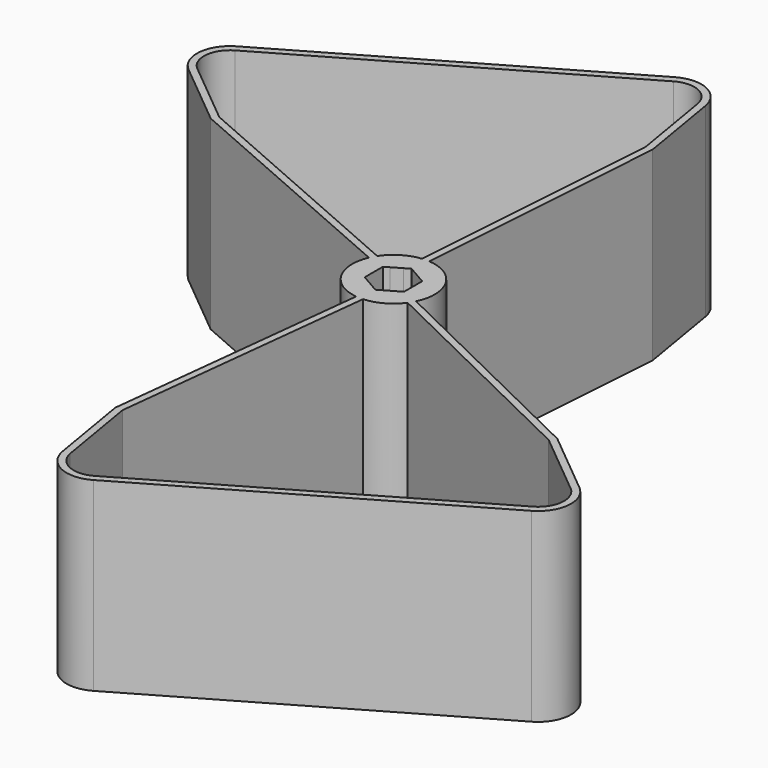
from build123d import *

# Parameters (mm, degrees)
F1_DEPTH = 22.5
F2_DEPTH = 22.5
F3_DEPTH = 21
F4_DEPTH = 1


# Not quite as in the source:
# - a feature names something its author has since deleted; it is built from what else it names


with BuildPart() as f1:
    # F0 (on Top) → F1 (new body, symmetric)
    with BuildSketch(Plane.XY):
        with BuildLine():
            Line((0.7049133584, 9.9751239169), (5.0995821323, 72.1634270217))
            Line((5.0995821323, 72.1634270217), (1.7099698283, 92.3552620466))
            ThreePointArc((1.7099698283, 92.3552620466), (-2.7689436701, 98.2673473553), (-10.179636045, 97.9590336386))
            Line((-10.179636045, 97.9590336386), (-82.8813710016, 55.9846673909))
            ThreePointArc((-82.8813710016, 55.9846673909), (-86.8537247, 49.720976393), (-83.9731653825, 42.8860808677))
            Line((-83.9731653825, 42.8860808677), (-68.1813294539, 29.8546729909))
            Line((-68.1813294539, 29.8546729909), (-9.1603226635, 4.0110458362))
            ThreePointArc((-9.1603226635, 4.0110458362), (-8.784741138, 4.7778994482), (-8.3451077857, 5.5099161558))
            Line((-8.3451077857, 5.5099161558), (-67.2822264653, 31.3168110829))
            Line((-67.2822264653, 31.3168110829), (-83.0737799078, 44.3479858524))
            ThreePointArc((-83.0737799078, 44.3479858524), (-85.1427917644, 49.7044488576), (-82.0166193538, 54.5210401885))
            Line((-82.0166193538, 54.5210401885), (-9.2869651685, 96.4475473538))
            ThreePointArc((-9.2869651685, 96.4475473538), (-3.5761256796, 96.734734482), (0, 92.2729535329))
            Line((0, 92.2729535329), (3.3895516703, 72.0814797017))
            Line((3.3895516703, 72.0814797017), (-1.0011183824, 9.9497619059))
            ThreePointArc((-1.0011183824, 9.9497619059), (-0.1486444145, 9.9988951809), (0.7049133584, 9.9751239169))
        make_face()
        with BuildLine():
            ThreePointArc((-9.1603226635, 4.0110458362), (-9.9846369617, -0.554098134), (-8.6602540378, -5))
            Line((-8.6602540378, -5), (-4.7631397208, -2.75))
            Line((-4.7631397208, -2.75), (-4.7631397208, 2.0856439719))
            Line((-4.7631397208, 2.0856439719), (-9.1603226635, 4.0110458362))
        make_face()
        with BuildLine():
            Line((4.7631397208, 2.75), (8.6602540378, 5))
            ThreePointArc((8.6602540378, 5), (5.3023159645, 8.4785284934), (0.7049133584, 9.9751239169))
            Line((0.7049133584, 9.9751239169), (0.373433245, 5.2843982155))
            Line((0.373433245, 5.2843982155), (4.7631397208, 2.75))
        make_face()
        with BuildLine():
            Line((-1.3715281953, 4.7081478273), (-1.0011183824, 9.9497619059))
            ThreePointArc((-1.0011183824, 9.9497619059), (-5.1735909645, 8.5576840636), (-8.3451077857, 5.5099161558))
            Line((-8.3451077857, 5.5099161558), (-3.589530539, 3.4275835771))
            Line((-3.589530539, 3.4275835771), (-1.3715281953, 4.7081478273))
        make_face()
        with BuildLine():
            Line((0.373433245, 5.2843982155), (0.7049133584, 9.9751239169))
            ThreePointArc((0.7049133584, 9.9751239169), (-0.1486444145, 9.9988951809), (-1.0011183824, 9.9497619059))
            Line((-1.0011183824, 9.9497619059), (-1.3715281953, 4.7081478273))
            Line((-1.3715281953, 4.7081478273), (0, 5.5))
            Line((0, 5.5), (0.373433245, 5.2843982155))
        make_face()
        with BuildLine():
            ThreePointArc((-8.3451077857, 5.5099161558), (-8.784741138, 4.7778994482), (-9.1603226635, 4.0110458362))
            Line((-9.1603226635, 4.0110458362), (-4.7631397208, 2.0856439719))
            Line((-4.7631397208, 2.0856439719), (-4.7631397208, 2.75))
            Line((-4.7631397208, 2.75), (-3.589530539, 3.4275835771))
            Line((-3.589530539, 3.4275835771), (-8.3451077857, 5.5099161558))
        make_face()
        with BuildLine():
            ThreePointArc((-8.3451077857, 5.5099161558), (-5.1735909645, 8.5576840636), (-1.0011183824, 9.9497619059))
            Line((-1.0011183824, 9.9497619059), (3.3895516703, 72.0814797017))
            Line((3.3895516703, 72.0814797017), (0, 92.2729535329))
            ThreePointArc((0, 92.2729535329), (-3.5761256796, 96.734734482), (-9.2869651685, 96.4475473538))
            Line((-9.2869651685, 96.4475473538), (-82.0166193538, 54.5210401885))
            ThreePointArc((-82.0166193538, 54.5210401885), (-85.1427917644, 49.7044488576), (-83.0737799078, 44.3479858524))
            Line((-83.0737799078, 44.3479858524), (-67.2822264653, 31.3168110829))
            Line((-67.2822264653, 31.3168110829), (-8.3451077857, 5.5099161558))
        make_face()
    extrude(amount=F1_DEPTH, both=True)

    # F0 (on Top) → F2 (cut, through all)
    with BuildSketch(Plane.XY):
        with BuildLine():
            ThreePointArc((-8.3451077857, 5.5099161558), (-5.1735909645, 8.5576840636), (-1.0011183824, 9.9497619059))
            Line((-1.0011183824, 9.9497619059), (3.3895516703, 72.0814797017))
            Line((3.3895516703, 72.0814797017), (0, 92.2729535329))
            ThreePointArc((0, 92.2729535329), (-3.5761256796, 96.734734482), (-9.2869651685, 96.4475473538))
            Line((-9.2869651685, 96.4475473538), (-82.0166193538, 54.5210401885))
            ThreePointArc((-82.0166193538, 54.5210401885), (-85.1427917644, 49.7044488576), (-83.0737799078, 44.3479858524))
            Line((-83.0737799078, 44.3479858524), (-67.2822264653, 31.3168110829))
            Line((-67.2822264653, 31.3168110829), (-8.3451077857, 5.5099161558))
        make_face()
    extrude(amount=F2_DEPTH, mode=Mode.SUBTRACT)

    # F0 (on Top) → F3 (cut)
    with BuildSketch(Plane.XY):
        with BuildLine():
            ThreePointArc((-8.3451077857, 5.5099161558), (-5.1735909645, 8.5576840636), (-1.0011183824, 9.9497619059))
            Line((-1.0011183824, 9.9497619059), (3.3895516703, 72.0814797017))
            Line((3.3895516703, 72.0814797017), (0, 92.2729535329))
            ThreePointArc((0, 92.2729535329), (-3.5761256796, 96.734734482), (-9.2869651685, 96.4475473538))
            Line((-9.2869651685, 96.4475473538), (-82.0166193538, 54.5210401885))
            ThreePointArc((-82.0166193538, 54.5210401885), (-85.1427917644, 49.7044488576), (-83.0737799078, 44.3479858524))
            Line((-83.0737799078, 44.3479858524), (-67.2822264653, 31.3168110829))
            Line((-67.2822264653, 31.3168110829), (-8.3451077857, 5.5099161558))
        make_face()
    extrude(amount=-F3_DEPTH, mode=Mode.SUBTRACT)

    # F0 (on Top) → F4 (join, symmetric)
    with BuildSketch(Plane.XY):
        Polygon((-4.7631397208, 2.0856439719), (0, 0), (0.373433245, 5.2843982155), (0, 5.5), (-1.3715281953, 4.7081478273), (-3.589530539, 3.4275835771), (-4.7631397208, 2.75), align=None)
        Polygon((0, 0), (4.7631397208, 2.75), (0.373433245, 5.2843982155), align=None)
        Polygon((-4.7631397208, 2.0856439719), (-4.7631397208, -2.75), (0, 0), align=None)
    extrude(amount=F4_DEPTH, both=True)

    # F5: F1 across face


with BuildPart() as f1_1:
    add(f1.part)
    add(f1.part.mirror(Plane(origin=(0, 0, 0), x_dir=(0.8660254038, 0.5, 0), z_dir=(0.5, -0.8660254038, 0))))


solid = f1_1.part
